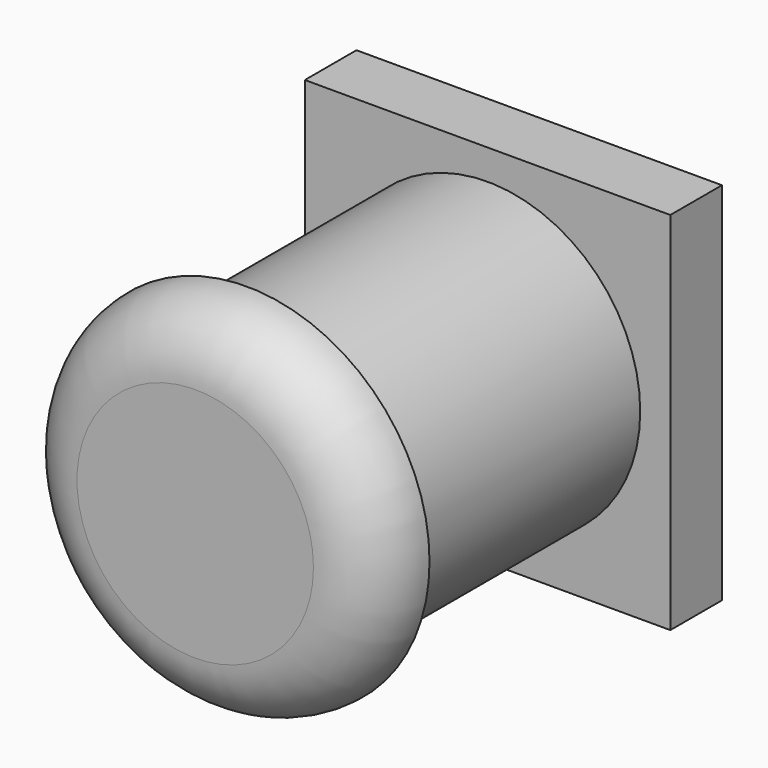
from build123d import *

# Parameters (mm, degrees)
F0_R     = 7.1
F1_DEPTH = 14
F2_R     = 8.5
F2_R_2   = 7.1
F3_DEPTH = 3
F4_R     = 2.99999
F5_W     = 17
F5_H     = 17
F5_R     = 7.1
F6_DEPTH = 3


# Not quite as in the source:
# - a fillet or chamfer is up to 0.001 mm smaller than in the source, because OpenCascade refuses the exact size


with BuildPart() as f1:
    # F0 (on Front) → F1 (new body)
    with BuildSketch(Plane.XZ):
        Circle(F0_R)
    extrude(amount=F1_DEPTH)

    # F2 (on face) → F3 (join)
    with BuildSketch(Plane.XZ.offset(14)):
        Circle(F2_R)
        Circle(F2_R_2, mode=Mode.SUBTRACT)
        Circle(F2_R_2)
    extrude(amount=F3_DEPTH)

    # F4 (radius 3 in the source; OpenCascade refuses exactly that, so slightly less here)
    f4_edges = [f1.edges().sort_by_distance(p)[0] for p in [
        (-8.5, -17, 0),
    ]]
    fillet(f4_edges, radius=F4_R)

    # F5 (on face) → F6 (join)
    with BuildSketch(Plane(origin=(0, 0, 0), x_dir=(-1, 0, 0), z_dir=(0, 1, 0))):
        with Locations((2.794e-06, 0)):
            Rectangle(F5_W, F5_H)
        Circle(F5_R, mode=Mode.SUBTRACT)
        Circle(F5_R)
    extrude(amount=F6_DEPTH)


solid = f1.part
